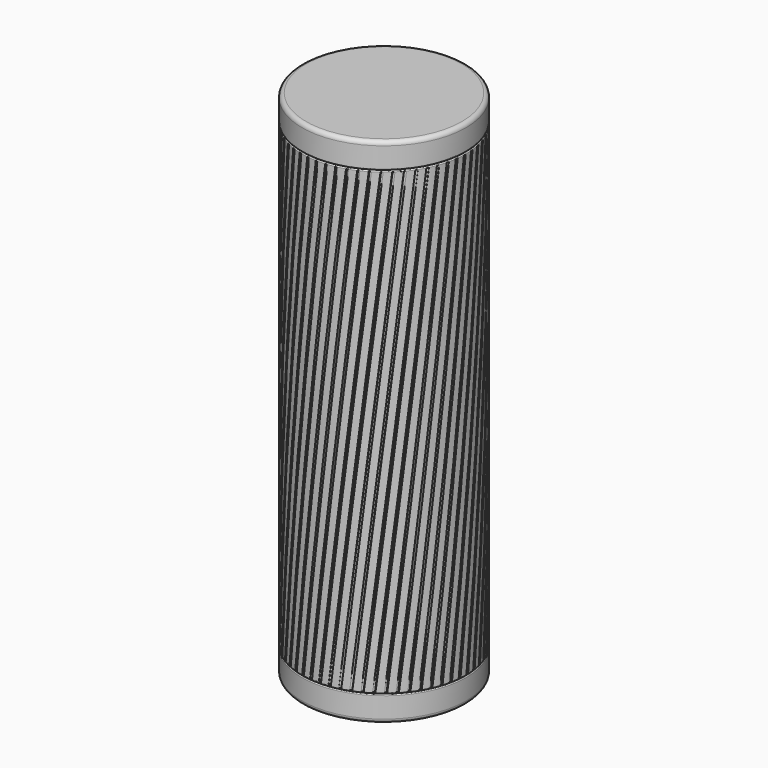
from build123d import *

# Parameters (mm, degrees)
F5_R             = 0.2
F5_2_R           = 0.2
F6_R             = 0.8
F10_DEPTH        = 10
F10_COPIES_COUNT = 56


# Not quite as in the source:
# - two fillets or chamfers of one size are made in one step
# - a pattern or mirror of a feature is missing from the dataset's text; its kind, count and spacing are read off the source's solid


with BuildPart() as f1:
    # F0 (on Front) → F1 (revolve)
    with BuildSketch(Plane.XZ):
        Polygon((0, 100), (0, 0), (16, 0), (16, 5), (13, 5), (13, 95), (16, 95), (16, 100), align=None)
    revolve(axis=Axis((0, 0, 50), (0, 0, 1)))

    # F5
    f5_edges = [f1.edges().sort_by_distance(p)[0] for p in [
        (-16, 0, 5),
        (-16, 0, 95),
    ]]
    fillet(f5_edges, radius=F5_R)

    # F6
    f6_edges = [f1.edges().sort_by_distance(p)[0] for p in [
        (-16, 0, 100),
        (-16, 0, 0),
    ]]
    fillet(f6_edges, radius=F6_R)


with BuildPart() as f4:
    # F2 (on Front) → F4 (revolve)
    with BuildSketch(Plane.XZ):
        Polygon((16, 91.9), (16, 94.9), (13.1, 94.9), (13.1, 5.1), (16, 5.1), (16, 8.1), align=None)
    revolve(axis=Axis((0, 0, 6.2946933322), (0, 0, 1)))

    # F5#2
    f5_2_edges = [f4.edges().sort_by_distance(p)[0] for p in [
        (-16, 0, 5.1),
        (-16, 0, 94.9),
    ]]
    fillet(f5_2_edges, radius=F5_2_R)

    # F9 (on offset) → F10 (cut)
    with BuildSketch(Plane.XZ.offset(25)):
        Polygon((5, 94.7), (-5, 5.3), (-4.7987526945, 5.3), (5.2012473055, 94.7), align=None)
        Polygon((4.7987526945, 94.7), (-5.2012473055, 5.3), (-5, 5.3), (5, 94.7), align=None)
    f10 = extrude(amount=-F10_DEPTH, mode=Mode.SUBTRACT)

    # F10_copies: F10 ×56 about axis
    f10_copies_axis = Axis((0, 0, 0), (0, 0, 1))
    for i in range(1, F10_COPIES_COUNT):
        add(f10.rotate(f10_copies_axis, i * 360 / F10_COPIES_COUNT), mode=Mode.SUBTRACT)


solid = Compound([f1.part, f4.part])
